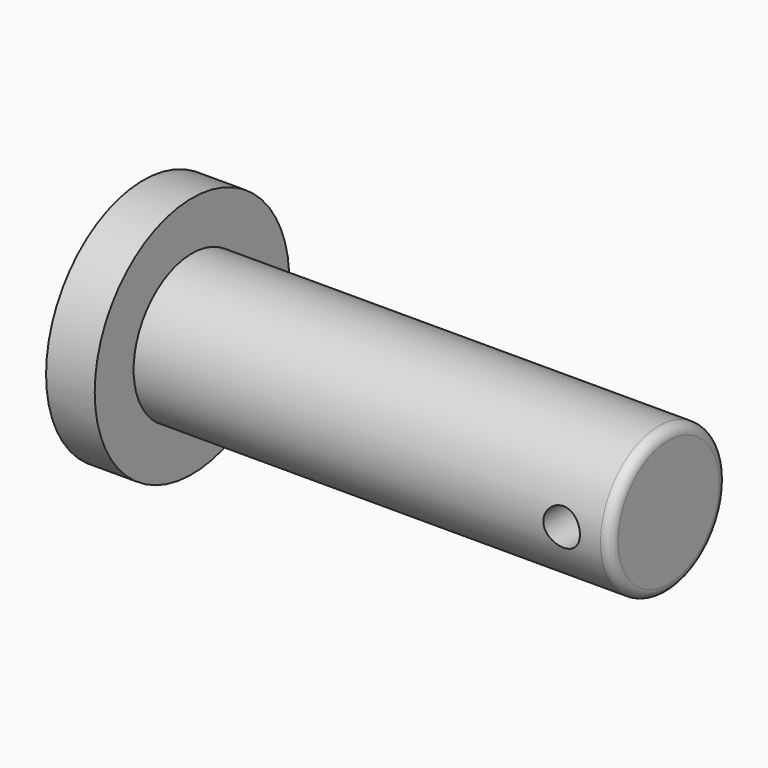
from build123d import *

# Parameters (mm, degrees)
F0_R     = 9.525
F1_DEPTH = 62.23
F3_R     = 2.3876
F4_DEPTH = 20.194
F5_R     = 15.875
F5_R_2   = 9.525
F6_DEPTH = 6.35
F7_R     = 1.27


with BuildPart() as f1:
    # F0 (on Right) → F1 (new body)
    with BuildSketch(Plane.YZ):
        Circle(F0_R)
    extrude(amount=F1_DEPTH)

    # F3 (on offset) → F4 (cut, through all)
    with BuildSketch(Plane.XZ.offset(10.668)):
        with Locations((55.88, 0)):
            Circle(F3_R)
    extrude(amount=-F4_DEPTH, mode=Mode.SUBTRACT)

    # F5 (on face) → F6 (join)
    with BuildSketch(Plane(origin=(0, 0, 0), x_dir=(0, -1, 0), z_dir=(-1, 0, 0))):
        Circle(F5_R)
        Circle(F5_R_2, mode=Mode.SUBTRACT)
        Circle(F5_R_2)
    extrude(amount=F6_DEPTH)

    # F7
    f7_edges = [f1.edges().sort_by_distance(p)[0] for p in [
        (62.23, -9.525, 0),
    ]]
    fillet(f7_edges, radius=F7_R)


solid = f1.part
